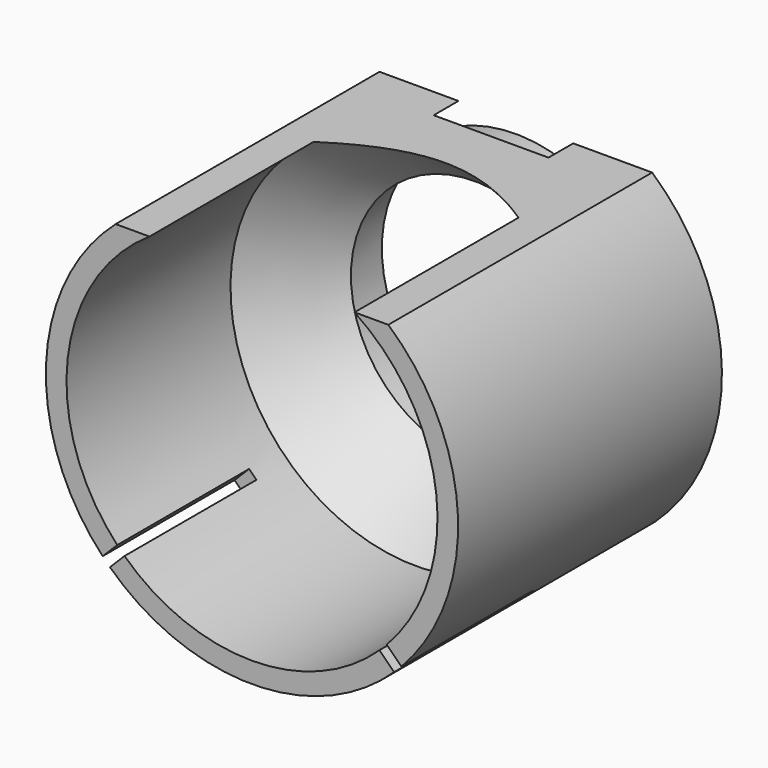
from build123d import *

# Parameters (mm, degrees)
F3_DEPTH = 8
F5_DEPTH = 16.001


with BuildPart() as f1:
    # F0 (on Top) → F1 (revolve)
    with BuildSketch(Plane.XY):
        Polygon((9, 0), (10, 0), (10, 16), (8, 16), (8, 14.5), (7, 14.5), (7, 16), (6.5, 16), (6.5, 13.5), (6, 13.5), (9, 9.9451635033), align=None)
    revolve(axis=Axis((0, 8.0098584294, 0), (0, 1, 0)))

    # F2 (on face) → F3 (cut)
    with BuildSketch(Plane.XZ):
        with BuildLine():
            Line((-6.8920810625, -7.2456344531), (-6.1847286297, -6.5382820203))
            ThreePointArc((-6.1847286297, -6.5382820203), (-6.3639610307, -6.3639610307), (-6.5382820203, -6.1847286297))
            Line((-6.5382820203, -6.1847286297), (-7.2456344531, -6.8920810625))
            ThreePointArc((-7.2456344531, -6.8920810625), (-7.0710678119, -7.0710678119), (-6.8920810625, -7.2456344531))
        make_face()
        with BuildLine():
            Line((7.2454194103, -6.8923071296), (6.5380675904, -6.1849553097))
            ThreePointArc((6.5380675904, -6.1849553097), (6.3639610307, -6.3639610307), (6.1849553097, -6.5380675904))
            Line((6.1849553097, -6.5380675904), (6.8923071296, -7.2454194103))
            ThreePointArc((6.8923071296, -7.2454194103), (7.0710678119, -7.0710678119), (7.2454194103, -6.8923071296))
        make_face()
    extrude(amount=-F3_DEPTH, mode=Mode.SUBTRACT)

    # F4 (on face) → F5 (cut, through all)
    with BuildSketch(Plane.XZ):
        with BuildLine():
            Line((-4.9749371855, 7.5), (0, 7.5))
            Line((0, 7.5), (4.9749371855, 7.5))
            ThreePointArc((4.9749371855, 7.5), (0, 9), (-4.9749371855, 7.5))
        make_face()
        with BuildLine():
            ThreePointArc((-4.9749371855, 7.5), (0, 9), (4.9749371855, 7.5))
            Line((4.9749371855, 7.5), (6.6143782777, 7.5))
            ThreePointArc((6.6143782777, 7.5), (0, 10), (-6.6143782777, 7.5))
            Line((-6.6143782777, 7.5), (-4.9749371855, 7.5))
        make_face()
    extrude(amount=-F5_DEPTH, mode=Mode.SUBTRACT)


solid = f1.part
